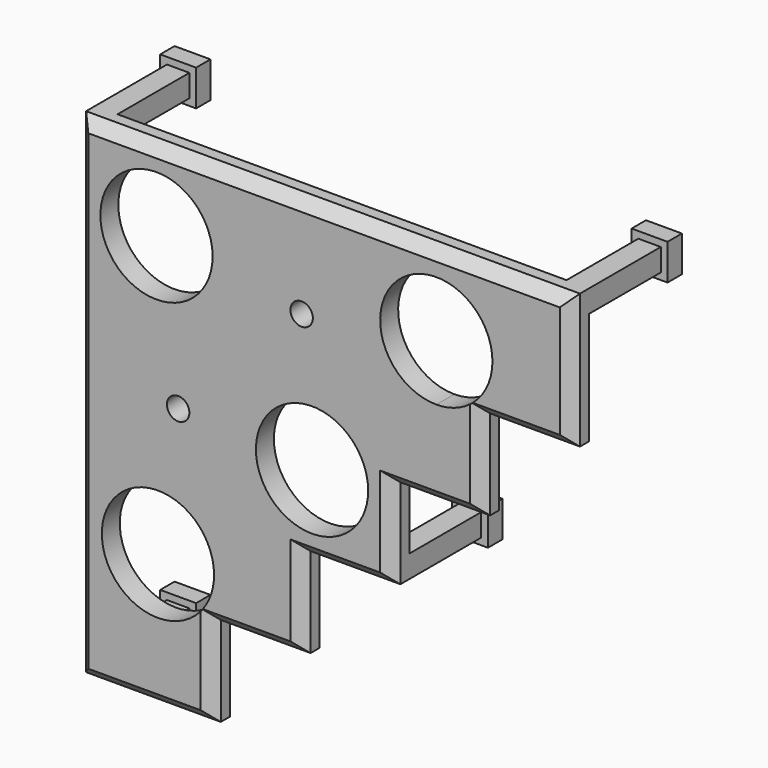
from build123d import *

# Parameters (mm, degrees)
F1_DEPTH  = 6.35
F3_SIZE   = 3.175
F5_W      = 6.35
F5_H      = 6.35
F6_DEPTH  = 25.4
F2_R      = 15.875
F7_DEPTH  = 25.4
F8_W      = 10.16
F8_H      = 10.16
F8_W_2    = 6.35
F8_H_2    = 6.35
F9_DEPTH  = 5.08
F10_W     = 10.16
F10_H     = 10.16
F10_W_2   = 6.35
F10_H_2   = 6.35
F11_DEPTH = 5.08
F12_W     = 10.16
F12_H     = 10.16
F12_W_2   = 6.35
F12_H_2   = 6.35
F13_DEPTH = 5.08
F14_W     = 10.16
F14_H     = 10.16
F14_W_2   = 6.35
F14_H_2   = 6.35
F15_DEPTH = 5.08
F4_R      = 3.175
F16_DEPTH = 25.4


# Not quite as in the source:
# - a feature names something its author has since deleted; it is built from what else it names


with BuildPart() as f1:
    # F0 (on Front) → F1 (new body)
    with BuildSketch(Plane.XZ):
        Polygon((139.7, 0), (0, 0), (0, -139.7), (38.1, -139.7), (38.1, -114.3), (63.5, -114.3), (63.5, -88.9), (88.9, -88.9), (88.9, -63.5), (114.3, -63.5), (114.3, -38.1), (139.7, -38.1), align=None)
    extrude(amount=F1_DEPTH)

    # F3
    f3_edges = [f1.edges().sort_by_distance(p)[0] for p in [
        (69.85, -6.35, 0),
        (0, -6.35, -69.85),
        (19.05, -6.35, -139.7),
        (38.1, -6.35, -127),
        (50.8, -6.35, -114.3),
        (63.5, -6.35, -101.6),
        (76.2, -6.35, -88.9),
        (88.9, -6.35, -76.2),
        (101.6, -6.35, -63.5),
        (114.3, -6.35, -50.8),
        (127, -6.35, -38.1),
        (139.7, -6.35, -19.05),
    ]]
    chamfer(f3_edges, length=F3_SIZE)

    # F5 (on face) → F6 (join)
    with BuildSketch(Plane(origin=(0, 0, 0), x_dir=(-1, 0, 0), z_dir=(0, 1, 0))):
        with Locations((-3.175, -3.175)):
            Rectangle(F5_W, F5_H)
        with Locations((-3.175, -136.525)):
            Rectangle(F5_W, F5_H)
        with Locations((-85.725, -85.725)):
            Rectangle(F5_W, F5_H)
        with Locations((-136.525, -3.175)):
            Rectangle(F5_W, F5_H)
    extrude(amount=F6_DEPTH)

    # F2 (on face) → F7 (cut)
    with BuildSketch(Plane.XZ.offset(6.35)):
        with BuildLine():
            ThreePointArc((117.475, -22.86), (90.3746798487, -11.6346798487), (101.6, -38.735))
            Line((101.6, -38.735), (101.6, -22.86))
            Line((101.6, -22.86), (117.475, -22.86))
        make_face()
        with BuildLine():
            Line((101.6, -22.86), (101.6, -38.735))
            ThreePointArc((101.6, -38.735), (112.8253201513, -34.0853201513), (117.475, -22.86))
            Line((117.475, -22.86), (101.6, -22.86))
        make_face()
        with BuildLine():
            ThreePointArc((82.3243596973, -66.4493596973), (51.7827721187, -60.3742602085), (77.6746798487, -77.6746798487))
            ThreePointArc((77.6746798487, -77.6746798487), (81.1159472759, -72.5244591861), (82.3243596973, -66.4493596973))
        make_face()
        with Locations((22.86, -101.6)):
            Circle(F2_R)
        with BuildLine():
            ThreePointArc((38.3256403027, -22.4506403027), (28.5257397915, -7.7840527241), (11.2253201513, -11.2253201513))
            ThreePointArc((11.2253201513, -11.2253201513), (16.3755408139, -37.1172278813), (38.3256403027, -22.4506403027))
        make_face()
    extrude(amount=-F7_DEPTH, mode=Mode.SUBTRACT)

    # F8 (on face) → F9 (join)
    with BuildSketch(Plane(origin=(0, 25.4, 0), x_dir=(-1, 0, 0), z_dir=(0, 1, 0))):
        with Locations((-3.175, -3.175)):
            Rectangle(F8_W, F8_H)
        with Locations((-3.175, -3.175)):
            Rectangle(F8_W_2, F8_H_2, mode=Mode.SUBTRACT)
        with Locations((-3.175, -3.175)):
            Rectangle(F8_W_2, F8_H_2)
    extrude(amount=F9_DEPTH)

    # F10 (on face) → F11 (join)
    with BuildSketch(Plane(origin=(0, 25.4, 0), x_dir=(-1, 0, 0), z_dir=(0, 1, 0))):
        with Locations((-136.525, -3.175)):
            Rectangle(F10_W, F10_H)
        with Locations((-136.525, -3.175)):
            Rectangle(F10_W_2, F10_H_2, mode=Mode.SUBTRACT)
        with Locations((-136.525, -3.175)):
            Rectangle(F10_W_2, F10_H_2)
    extrude(amount=F11_DEPTH)

    # F12 (on face) → F13 (join)
    with BuildSketch(Plane(origin=(0, 25.4, 0), x_dir=(-1, 0, 0), z_dir=(0, 1, 0))):
        with Locations((-85.725, -85.725)):
            Rectangle(F12_W, F12_H)
        with Locations((-85.725, -85.725)):
            Rectangle(F12_W_2, F12_H_2, mode=Mode.SUBTRACT)
        with Locations((-85.725, -85.725)):
            Rectangle(F12_W_2, F12_H_2)
    extrude(amount=F13_DEPTH)

    # F14 (on face) → F15 (join)
    with BuildSketch(Plane(origin=(0, 25.4, 0), x_dir=(-1, 0, 0), z_dir=(0, 1, 0))):
        with Locations((-3.175, -136.525)):
            Rectangle(F14_W, F14_H)
        with Locations((-3.175, -136.525)):
            Rectangle(F14_W_2, F14_H_2, mode=Mode.SUBTRACT)
        with Locations((-3.175, -136.525)):
            Rectangle(F14_W_2, F14_H_2)
    extrude(amount=F15_DEPTH)

    # F4 (on face) → F16 (cut)
    with BuildSketch(Plane.XZ.offset(6.35)):
        with Locations((63.5, -28.575)):
            Circle(F4_R)
        with Locations((28.575, -63.5)):
            Circle(F4_R)
    extrude(amount=-F16_DEPTH, mode=Mode.SUBTRACT)


solid = f1.part
